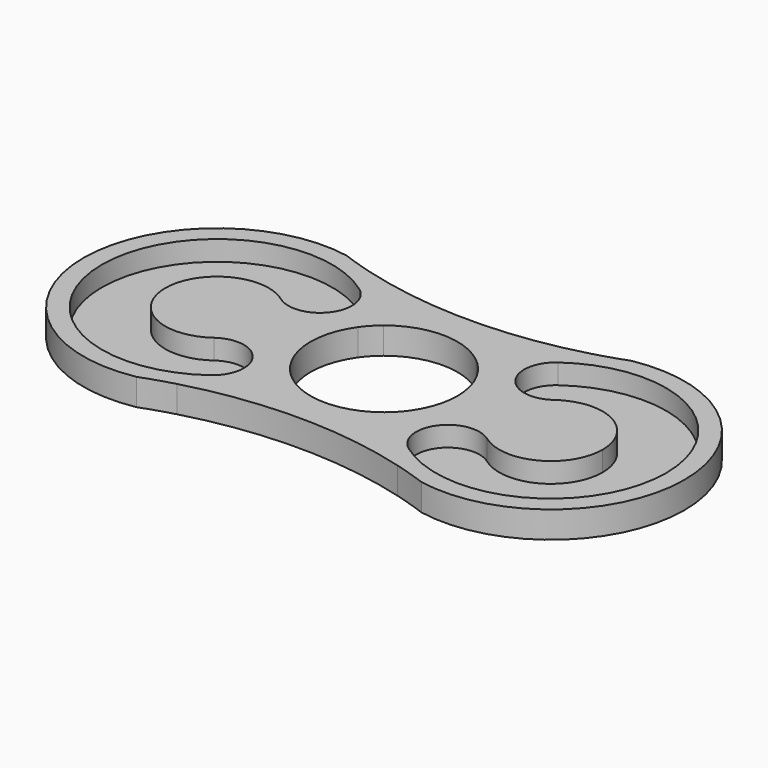
from build123d import *

# Parameters (mm, degrees)
F1_DEPTH = 4
F2_DEPTH = 1


with BuildPart() as f1:
    # F0 (on Top) → F1 (new body)
    with BuildSketch(Plane.XY):
        with BuildLine():
            ThreePointArc((33.96875, 44.7240123715), (35.4798914594, 41.6976549267), (36, 38.3552194374))
            ThreePointArc((36, 38.3552194374), (35.4798914594, 35.0127839481), (33.96875, 31.9864265033))
            ThreePointArc((33.96875, 31.9864265033), (34.890304672, 30.0329837344), (36.04875, 28.2100174464))
            ThreePointArc((36.04875, 28.2100174464), (38.9773253879, 32.9114730252), (40, 38.3552194374))
            ThreePointArc((40, 38.3552194374), (38.9773253879, 43.7989658495), (36.04875, 48.5004214283))
            ThreePointArc((36.04875, 48.5004214283), (34.890304672, 46.6774551404), (33.96875, 44.7240123715))
        make_face()
        with BuildLine():
            ThreePointArc((31.92, 46.9058685355), (33.0189287452, 45.8849459782), (33.96875, 44.7240123715))
            ThreePointArc((33.96875, 44.7240123715), (34.890304672, 46.6774551404), (36.04875, 48.5004214283))
            ThreePointArc((36.04875, 48.5004214283), (35.0671824784, 49.4751041915), (34, 50.3552194374))
            ThreePointArc((34, 50.3552194374), (32.8729423014, 48.6830408238), (31.92, 46.9058685355))
        make_face()
        with BuildLine():
            ThreePointArc((36.04875, 28.2100174464), (34.890304672, 30.0329837344), (33.96875, 31.9864265033))
            ThreePointArc((33.96875, 31.9864265033), (33.0189287452, 30.8254928966), (31.92, 29.8045703392))
            ThreePointArc((31.92, 29.8045703392), (32.8729423014, 28.027398051), (34, 26.3552194374))
            ThreePointArc((34, 26.3552194374), (35.0671824784, 27.2353346832), (36.04875, 28.2100174464))
        make_face()
        with BuildLine():
            ThreePointArc((18.08, 46.9058685355), (25, 49.3552194374), (31.92, 46.9058685355))
            ThreePointArc((31.92, 46.9058685355), (32.8729423014, 48.6830408238), (34, 50.3552194374))
            ThreePointArc((34, 50.3552194374), (25, 53.3552194374), (16, 50.3552194374))
            ThreePointArc((16, 50.3552194374), (17.1270576986, 48.6830408238), (18.08, 46.9058685355))
        make_face()
        with BuildLine():
            ThreePointArc((39.8607042186, 52.31076246), (37.804989803, 50.5553926449), (36.04875, 48.5004214283))
            ThreePointArc((36.04875, 48.5004214283), (38.9773253879, 43.7989658495), (40, 38.3552194374))
            ThreePointArc((40, 38.3552194374), (38.9773253879, 32.9114730252), (36.04875, 28.2100174464))
            ThreePointArc((36.04875, 28.2100174464), (37.8049899077, 26.1550461251), (39.8607044582, 24.3996762406))
            ThreePointArc((39.8607044582, 24.3996762406), (38.8098535793, 31.0344868958), (45.4446642345, 32.0853377748))
            ThreePointArc((45.4446642345, 32.0853377748), (42.25, 38.3552195837), (45.4446644712, 44.625101272))
            ThreePointArc((45.4446644712, 44.625101272), (38.8098537523, 45.6759517408), (39.8607042186, 52.31076246))
        make_face()
        with BuildLine():
            ThreePointArc((34, 50.3552194374), (35.0671824784, 49.4751041915), (36.04875, 48.5004214283))
            ThreePointArc((36.04875, 48.5004214283), (37.804989803, 50.5553926449), (39.8607042186, 52.31076246))
            ThreePointArc((39.8607042186, 52.31076246), (57.8313360218, 53.7250820299), (67.25, 38.3552194374))
            ThreePointArc((67.25, 38.3552194374), (57.8313361537, 22.985356912), (39.8607044582, 24.3996762406))
            ThreePointArc((39.8607044582, 24.3996762406), (37.8049899077, 26.1550461251), (36.04875, 28.2100174464))
            ThreePointArc((36.04875, 28.2100174464), (35.0671824784, 27.2353346832), (34, 26.3552194374))
            ThreePointArc((34, 26.3552194374), (37.3874296651, 22.8335227019), (41.5277360562, 20.2383559211))
            ThreePointArc((41.5277360562, 20.2383559211), (43.9514682435, 19.5144497823), (46.3436548255, 18.6922812041))
            ThreePointArc((46.3436548255, 18.6922812041), (62.7842304522, 22.9746000823), (70, 38.3552194374))
            ThreePointArc((70, 38.3552194374), (62.7842304522, 53.7358387924), (46.3436548255, 58.0181576706))
            ThreePointArc((46.3436548255, 58.0181576706), (43.9514682435, 57.1959890924), (41.5277360562, 56.4720829536))
            ThreePointArc((41.5277360562, 56.4720829536), (37.3874296651, 53.8769161728), (34, 50.3552194374))
        make_face()
        with BuildLine():
            ThreePointArc((34, 26.3552194374), (32.8729423014, 28.027398051), (31.92, 29.8045703392))
            ThreePointArc((31.92, 29.8045703392), (25, 27.3552194374), (18.08, 29.8045703392))
            ThreePointArc((18.08, 29.8045703392), (17.1270576986, 28.027398051), (16, 26.3552194374))
            ThreePointArc((16, 26.3552194374), (25, 23.3552194374), (34, 26.3552194374))
        make_face()
        with BuildLine():
            ThreePointArc((16.03125, 44.7240123715), (16.9810712548, 45.8849459782), (18.08, 46.9058685355))
            ThreePointArc((18.08, 46.9058685355), (17.1270576986, 48.6830408238), (16, 50.3552194374))
            ThreePointArc((16, 50.3552194374), (14.9328175216, 49.4751041915), (13.95125, 48.5004214283))
            ThreePointArc((13.95125, 48.5004214283), (15.109695328, 46.6774551404), (16.03125, 44.7240123715))
        make_face()
        with BuildLine():
            ThreePointArc((16, 50.3552194374), (25, 53.3552194374), (34, 50.3552194374))
            ThreePointArc((34, 50.3552194374), (37.3874296651, 53.8769161728), (41.5277360562, 56.4720829536))
            ThreePointArc((41.5277360562, 56.4720829536), (25, 54.228538177), (8.4722639438, 56.4720829536))
            ThreePointArc((8.4722639438, 56.4720829536), (12.6125703349, 53.8769161728), (16, 50.3552194374))
        make_face()
        with BuildLine():
            ThreePointArc((16, 26.3552194374), (17.1270576986, 28.027398051), (18.08, 29.8045703392))
            ThreePointArc((18.08, 29.8045703392), (16.9810712548, 30.8254928966), (16.03125, 31.9864265033))
            ThreePointArc((16.03125, 31.9864265033), (15.109695328, 30.0329837344), (13.95125, 28.2100174464))
            ThreePointArc((13.95125, 28.2100174464), (14.9328175216, 27.2353346832), (16, 26.3552194374))
        make_face()
        with BuildLine():
            ThreePointArc((41.5277360562, 20.2383559211), (37.3874296651, 22.8335227019), (34, 26.3552194374))
            ThreePointArc((34, 26.3552194374), (25, 23.3552194374), (16, 26.3552194374))
            ThreePointArc((16, 26.3552194374), (12.6125703349, 22.8335227019), (8.4722639438, 20.2383559211))
            ThreePointArc((8.4722639438, 20.2383559211), (25, 22.4819006978), (41.5277360562, 20.2383559211))
        make_face()
        with BuildLine():
            ThreePointArc((16.03125, 31.9864265033), (14, 38.3552194374), (16.03125, 44.7240123715))
            ThreePointArc((16.03125, 44.7240123715), (15.109695328, 46.6774551404), (13.95125, 48.5004214283))
            ThreePointArc((13.95125, 48.5004214283), (10, 38.3552194374), (13.95125, 28.2100174464))
            ThreePointArc((13.95125, 28.2100174464), (15.109695328, 30.0329837344), (16.03125, 31.9864265033))
        make_face()
        with BuildLine():
            ThreePointArc((13.95125, 48.5004214283), (14.9328175216, 49.4751041915), (16, 50.3552194374))
            ThreePointArc((16, 50.3552194374), (12.6125703349, 53.8769161728), (8.4722639438, 56.4720829536))
            ThreePointArc((8.4722639438, 56.4720829536), (6.0485317565, 57.1959890924), (3.6563451745, 58.0181576706))
            ThreePointArc((3.6563451745, 58.0181576706), (-20, 38.3552194374), (3.6563451745, 18.6922812041))
            ThreePointArc((3.6563451745, 18.6922812041), (6.0485317565, 19.5144497823), (8.4722639438, 20.2383559211))
            ThreePointArc((8.4722639438, 20.2383559211), (12.6125703349, 22.8335227019), (16, 26.3552194374))
            ThreePointArc((16, 26.3552194374), (14.9328175216, 27.2353346832), (13.95125, 28.2100174464))
            ThreePointArc((13.95125, 28.2100174464), (12.1950101323, 26.1550461651), (10.1392956333, 24.3996763071))
            ThreePointArc((10.1392956333, 24.3996763071), (-17.25, 38.3552194393), (10.1392956365, 52.3107625653))
            ThreePointArc((10.1392956365, 52.3107625653), (12.1950101337, 50.5553927082), (13.95125, 48.5004214283))
        make_face()
        with BuildLine():
            ThreePointArc((50, 46.1052194374), (47.6051183973, 45.7259074724), (45.4446644712, 44.625101272))
            ThreePointArc((45.4446644712, 44.625101272), (42.25, 38.3552195837), (45.4446642345, 32.0853377748))
            ThreePointArc((45.4446642345, 32.0853377748), (53.5184263398, 31.449918858), (57.75, 38.3552194374))
            ThreePointArc((57.75, 38.3552194374), (55.4800775542, 43.8352969916), (50, 46.1052194374))
        make_face()
        with BuildLine():
            ThreePointArc((13.95125, 28.2100174464), (10, 38.3552194374), (13.95125, 48.5004214283))
            ThreePointArc((13.95125, 48.5004214283), (12.1950101337, 50.5553927082), (10.1392956365, 52.3107625653))
            ThreePointArc((10.1392956365, 52.3107625653), (11.5795966532, 50.6243867219), (12.0973156537, 48.4679318671))
            ThreePointArc((12.0973156537, 48.4679318671), (9.503770504, 44.2356508652), (4.5553356627, 44.6251011747))
            ThreePointArc((4.5553356627, 44.6251011747), (6.9053005505, 41.8736458338), (7.75, 38.3552194374))
            ThreePointArc((7.75, 38.3552194374), (6.9053005928, 34.8367931239), (4.5553358133, 32.0853378094))
            ThreePointArc((4.5553358133, 32.0853378094), (9.5037705869, 32.4747879673), (12.0973156537, 28.2425070077))
            ThreePointArc((12.0973156537, 28.2425070077), (11.5795966523, 26.0860521511), (10.1392956333, 24.3996763071))
            ThreePointArc((10.1392956333, 24.3996763071), (12.1950101323, 26.1550461651), (13.95125, 28.2100174464))
        make_face()
        with BuildLine():
            ThreePointArc((7.75, 38.3552194374), (6.9053005505, 41.8736458338), (4.5553356627, 44.6251011747))
            ThreePointArc((4.5553356627, 44.6251011747), (2.3948816814, 45.7259074468), (0, 46.1052194374))
            ThreePointArc((0, 46.1052194374), (-7.3706879807, 35.9603376675), (4.5553358133, 32.0853378094))
            ThreePointArc((4.5553358133, 32.0853378094), (6.9053005928, 34.8367931239), (7.75, 38.3552194374))
        make_face()
    extrude(amount=F1_DEPTH)

    # F0 (on Top) → F2 (join)
    with BuildSketch(Plane.XY):
        with BuildLine():
            ThreePointArc((67.25, 38.3552194374), (57.8313360218, 53.7250820299), (39.8607042186, 52.31076246))
            ThreePointArc((39.8607042186, 52.31076246), (44.8091391214, 52.7002129073), (47.4026843463, 48.4679318671))
            ThreePointArc((47.4026843463, 48.4679318671), (46.8849653857, 46.3114770905), (45.4446644712, 44.625101272))
            ThreePointArc((45.4446644712, 44.625101272), (47.6051183973, 45.7259074724), (50, 46.1052194374))
            ThreePointArc((50, 46.1052194374), (55.4800775542, 43.8352969916), (57.75, 38.3552194374))
            ThreePointArc((57.75, 38.3552194374), (53.5184263398, 31.449918858), (45.4446642345, 32.0853377748))
            ThreePointArc((45.4446642345, 32.0853377748), (46.8849653193, 30.3989619146), (47.4026843463, 28.2425070077))
            ThreePointArc((47.4026843463, 28.2425070077), (44.8091392533, 24.0102260347), (39.8607044582, 24.3996762406))
            ThreePointArc((39.8607044582, 24.3996762406), (57.8313361537, 22.985356912), (67.25, 38.3552194374))
        make_face()
        with BuildLine():
            ThreePointArc((47.4026843463, 48.4679318671), (44.8091391214, 52.7002129073), (39.8607042186, 52.31076246))
            ThreePointArc((39.8607042186, 52.31076246), (38.8098537523, 45.6759517408), (45.4446644712, 44.625101272))
            ThreePointArc((45.4446644712, 44.625101272), (46.8849653857, 46.3114770905), (47.4026843463, 48.4679318671))
        make_face()
        with BuildLine():
            ThreePointArc((45.4446642345, 32.0853377748), (38.8098535793, 31.0344868958), (39.8607044582, 24.3996762406))
            ThreePointArc((39.8607044582, 24.3996762406), (44.8091392533, 24.0102260347), (47.4026843463, 28.2425070077))
            ThreePointArc((47.4026843463, 28.2425070077), (46.8849653193, 30.3989619146), (45.4446642345, 32.0853377748))
        make_face()
        with BuildLine():
            ThreePointArc((4.5553356627, 44.6251011747), (3.5044849583, 51.2599118539), (10.1392956365, 52.3107625653))
            ThreePointArc((10.1392956365, 52.3107625653), (-17.25, 38.3552194393), (10.1392956333, 24.3996763071))
            ThreePointArc((10.1392956333, 24.3996763071), (3.5044849025, 25.4505270977), (4.5553358133, 32.0853378094))
            ThreePointArc((4.5553358133, 32.0853378094), (-7.3706879807, 35.9603376675), (0, 46.1052194374))
            ThreePointArc((0, 46.1052194374), (2.3948816814, 45.7259074468), (4.5553356627, 44.6251011747))
        make_face()
        with BuildLine():
            ThreePointArc((12.0973156537, 48.4679318671), (11.5795966532, 50.6243867219), (10.1392956365, 52.3107625653))
            ThreePointArc((10.1392956365, 52.3107625653), (3.5044849583, 51.2599118539), (4.5553356627, 44.6251011747))
            ThreePointArc((4.5553356627, 44.6251011747), (9.503770504, 44.2356508652), (12.0973156537, 48.4679318671))
        make_face()
        with BuildLine():
            ThreePointArc((4.5553358133, 32.0853378094), (3.5044849025, 25.4505270977), (10.1392956333, 24.3996763071))
            ThreePointArc((10.1392956333, 24.3996763071), (11.5795966523, 26.0860521511), (12.0973156537, 28.2425070077))
            ThreePointArc((12.0973156537, 28.2425070077), (9.5037705869, 32.4747879673), (4.5553358133, 32.0853378094))
        make_face()
    extrude(amount=F2_DEPTH)


solid = f1.part
